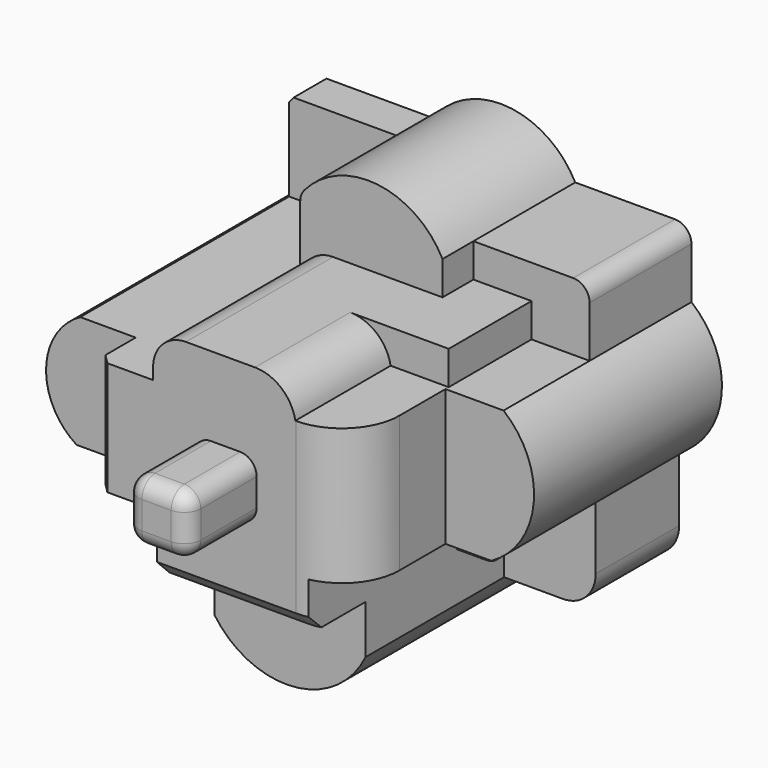
from build123d import *

# Parameters (mm, degrees)
F0_W         = 19.224062562
F0_H         = 18.6825376004
F1_DEPTH     = 134.874
F2_DEPTH     = 108.204
F0_W_2       = 18.3131638914
F0_H_2       = 18.7943680212
F3_DEPTH     = 83.058
F0_W_3       = 17.1565823257
F0_H_3       = 13.6970020831
F4_DEPTH     = 25.4
F0_W_4       = 17.9688669741
F0_H_4       = 10.4478634894
F5_DEPTH     = 71.374
F0_W_5       = 14.1782090068
F0_H_5       = 15.0508098304
F6_DEPTH     = 50.546
F7_DEPTH     = 72.644
F8_DEPTH     = 85.852
F9_DEPTH     = 51.308
F10_DEPTH    = 93.472
F11_DEPTH    = 61.214
F12_DEPTH    = 32.258
F13_DEPTH    = 39.37
F14_DEPTH    = 12.7
F15_R        = 5.08
F16_R        = 10.16
F17_R        = 5.08
F18_T1_DEPTH = 68.0767879487
F19_R        = 10.16
F20_SIZE     = 3.0226
F21_R        = 17.78
F22_SIZE     = 4.8203104
F23_R        = 5.08
F24_R        = 5.08
F25_R        = 5.08
F26_R        = 5.08
F27_R        = 5.08


# Not quite as in the source:
# - a fillet or chamfer that OpenCascade refuses, or shapes differently, is made with other operations: its cross-section is extruded or revolved along the edge and cut away or added


with BuildPart() as f1:
    # F0 (on Front) → F1 (new body)
    with BuildSketch(Plane.XZ):
        Rectangle(F0_W, F0_H)
    extrude(amount=F1_DEPTH)

    # F0 (on Front) → F2 (join)
    with BuildSketch(Plane.XZ):
        Polygon((-21.2547723204, -33.8216274977), (25.389727205, -33.8216274977), (25.389727205, -18.7708176672), (39.5679362118, -18.7708176672), (39.5679362118, 23.3737640083), (21.5990692377, 23.3737640083), (21.5990692377, 33.8216274977), (-22.4113538861, 33.8216274977), (-22.4113538861, 20.1246254146), (-39.5679362118, 20.1246254146), (-39.5679362118, -15.0272594765), (-21.2547723204, -15.0272594765), align=None)
        Rectangle(F0_W, F0_H, mode=Mode.SUBTRACT)
    extrude(amount=F2_DEPTH)

    # F0 (on Front) → F3 (join)
    with BuildSketch(Plane.XZ):
        with Locations((-30.4113542661, -24.4244434871)):
            Rectangle(F0_W_2, F0_H_2)
    extrude(amount=F3_DEPTH)

    # F0 (on Front) → F4 (join)
    with BuildSketch(Plane.XZ):
        with Locations((-30.989645049, 26.9731264561)):
            Rectangle(F0_W_3, F0_H_3)
    extrude(amount=F4_DEPTH)

    # F0 (on Front) → F5 (join)
    with BuildSketch(Plane.XZ):
        with Locations((30.5835027248, 28.597695753)):
            Rectangle(F0_W_4, F0_H_4)
    extrude(amount=F5_DEPTH)

    # F0 (on Front) → F6 (join)
    with BuildSketch(Plane.XZ):
        with Locations((32.4788317084, -26.2962225825)):
            Rectangle(F0_W_5, F0_H_5)
    extrude(amount=F6_DEPTH)

    # F0 (on Front) → F7 (join)
    with BuildSketch(Plane.XZ):
        with BuildLine():
            Line((39.5679362118, 23.3737640083), (39.5679362118, -18.7708176672))
            Line((39.5679362118, -18.7708176672), (53.7461452186, -18.7708176672))
            ThreePointArc((53.7461452186, -18.7708176672), (66.8748667644, 1.2910953871), (57.5368031859, 23.3737640083))
            Line((57.5368031859, 23.3737640083), (39.5679362118, 23.3737640083))
        make_face()
    extrude(amount=F7_DEPTH)

    # F0 (on Front) → F8 (join)
    with BuildSketch(Plane.XZ):
        with BuildLine():
            Line((25.389727205, -48.8724373281), (25.389727205, -33.8216274977))
            Line((25.389727205, -33.8216274977), (-21.2547723204, -33.8216274977))
            Line((-21.2547723204, -33.8216274977), (-21.2547723204, -52.6159955189))
            ThreePointArc((-21.2547723204, -52.6159955189), (3.1426231279, -64.1404640217), (25.389727205, -48.8724373281))
        make_face()
    extrude(amount=F8_DEPTH)

    # F0 (on Front) → F9 (join)
    with BuildSketch(Plane.XZ):
        with BuildLine():
            Line((-22.4113538861, 33.8216274977), (21.5990692377, 33.8216274977))
            Line((21.5990692377, 33.8216274977), (21.5990692377, 44.2694909871))
            ThreePointArc((21.5990692377, 44.2694909871), (0.4961178031, 58.1154072117), (-22.4113538861, 47.5186295807))
            Line((-22.4113538861, 47.5186295807), (-22.4113538861, 33.8216274977))
        make_face()
    extrude(amount=F9_DEPTH)

    # F0 (on Front) → F10 (join)
    with BuildSketch(Plane.XZ):
        with BuildLine():
            Line((-57.8811001033, -15.0272594765), (-39.5679362118, -15.0272594765))
            Line((-39.5679362118, -15.0272594765), (-39.5679362118, 20.1246254146))
            Line((-39.5679362118, 20.1246254146), (-56.7245185375, 20.1246254146))
            ThreePointArc((-56.7245185375, 20.1246254146), (-67.2856136398, 2.8771412434), (-57.8811001033, -15.0272594765))
        make_face()
    extrude(amount=F10_DEPTH)

    # F0 (on Front) → F11 (join)
    with BuildSketch(Plane.XZ):
        with BuildLine():
            Line((-21.2547723204, -52.6159955189), (-21.2547723204, -33.8216274977))
            Line((-21.2547723204, -33.8216274977), (-39.5679362118, -33.8216274977))
            Line((-39.5679362118, -33.8216274977), (-39.5679362118, -15.0272594765))
            Line((-39.5679362118, -15.0272594765), (-57.8811001033, -15.0272594765))
            Line((-57.8811001033, -15.0272594765), (-57.8811001033, -44.4008079084))
            ThreePointArc((-57.8811001033, -44.4008079084), (-54.3606128257, -48.647479537), (-50.5293034549, -52.6159955189))
            Line((-50.5293034549, -52.6159955189), (-21.2547723204, -52.6159955189))
        make_face()
    extrude(amount=F11_DEPTH)

    # F0 (on Front) → F12 (join)
    with BuildSketch(Plane.XZ):
        Polygon((39.5679362118, -18.7708176672), (39.5679362118, -33.8216274977), (25.389727205, -33.8216274977), (25.389727205, -48.8724373281), (53.7461452186, -48.8724373281), (53.7461452186, -18.7708176672), align=None)
    extrude(amount=F12_DEPTH)

    # F0 (on Front) → F13 (join)
    with BuildSketch(Plane.XZ):
        Polygon((39.5679362118, 33.8216274977), (39.5679362118, 23.3737640083), (57.5368031859, 23.3737640083), (57.5368031859, 44.2694909871), (21.5990692377, 44.2694909871), (21.5990692377, 33.8216274977), align=None)
    extrude(amount=F13_DEPTH)

    # F0 (on Front) → F14 (join)
    with BuildSketch(Plane.XZ):
        with BuildLine():
            Line((-56.7245185375, 20.1246254146), (-39.5679362118, 20.1246254146))
            Line((-39.5679362118, 20.1246254146), (-39.5679362118, 33.8216274977))
            Line((-39.5679362118, 33.8216274977), (-22.4113538861, 33.8216274977))
            Line((-22.4113538861, 33.8216274977), (-22.4113538861, 47.5186295807))
            Line((-22.4113538861, 47.5186295807), (-55.3500978757, 47.5186295807))
            ThreePointArc((-55.3500978757, 47.5186295807), (-56.0433767246, 46.6989659134), (-56.7245185375, 45.8691888828))
            Line((-56.7245185375, 45.8691888828), (-56.7245185375, 20.1246254146))
        make_face()
    extrude(amount=F14_DEPTH)

    # F15
    f15_edges = [f1.edges().sort_by_distance(p)[0] for p in [
        (57.536803, -19.685, 44.269491),
    ]]
    fillet(f15_edges, radius=F15_R)

    # F16
    f16_edges = [f1.edges().sort_by_distance(p)[0] for p in [
        (53.746145, -16.129, -48.872437),
    ]]
    fillet(f16_edges, radius=F16_R)

    # F17
    f17_edges = [f1.edges().sort_by_distance(p)[0] for p in [
        (39.567936, -41.402, -33.821627),
    ]]
    fillet(f17_edges, radius=F17_R)

    # F18: fillet of radius 12.7 on 1 edges, made by hand

    # F18_s2 → F18_t1 (cut)
    with BuildSketch(Plane.XZ.offset(71.374)):
        with BuildLine():
            ThreePointArc((21.5990692377, 23.3737640083), (17.2455325804, 30.8656547371), (9.1003540582, 33.8216274977))
            Line((9.1003540582, 33.8216274977), (21.5990692377, 33.8216274977))
            Line((21.5990692377, 33.8216274977), (21.5990692377, 23.3737640083))
        make_face()
    extrude(amount=F18_T1_DEPTH, mode=Mode.SUBTRACT)

    # F19
    f19_edges = [f1.edges().sort_by_distance(p)[0] for p in [
        (-22.411354, -79.756, 33.821627),
    ]]
    fillet(f19_edges, radius=F19_R)

    # F20
    f20_edges = [f1.edges().sort_by_distance(p)[0] for p in [
        (-39.567936, -72.136, -33.821627),
        (-39.567936, -108.204, 2.548683),
    ]]
    chamfer(f20_edges, length=F20_SIZE)

    # F21
    f21_edges = [f1.edges().sort_by_distance(p)[0] for p in [
        (39.567936, -108.204, 2.301473),
    ]]
    fillet(f21_edges, radius=F21_R)

    # F22
    f22_edges = [f1.edges().sort_by_distance(p)[0] for p in [
        (0.266582, -108.204, -33.821627),
        (23.59824, -108.1116, -33.821627),
    ]]
    chamfer(f22_edges, length=F22_SIZE)

    # F23
    f23_edges = [f1.edges().sort_by_distance(p)[0] for p in [
        (0, -134.874, -9.341269),
    ]]
    fillet(f23_edges, radius=F23_R)

    # F24
    f24_edges = [f1.edges().sort_by_distance(p)[0] for p in [
        (-9.612031, -134.874, 2.54),
    ]]
    fillet(f24_edges, radius=F24_R)

    # F25
    f25_edges = [f1.edges().sort_by_distance(p)[0] for p in [
        (2.54, -134.874, 9.341269),
    ]]
    fillet(f25_edges, radius=F25_R)

    # F26
    f26_edges = [f1.edges().sort_by_distance(p)[0] for p in [
        (9.612031, -134.874, 0),
    ]]
    fillet(f26_edges, radius=F26_R)

    # F27
    f27_edges = [f1.edges().sort_by_distance(p)[0] for p in [
        (-22.411354, -32.004, 47.51863),
    ]]
    fillet(f27_edges, radius=F27_R)


solid = f1.part
